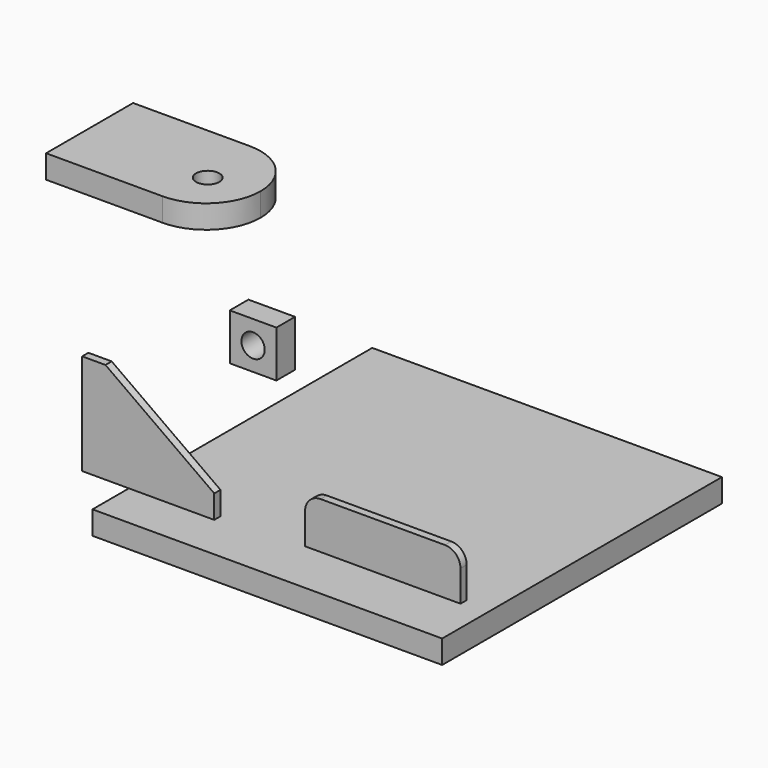
from build123d import *

# Parameters (mm, degrees)
F1_DEPTH  = 6.35
F0_W      = 127
F0_H      = 38.1
F2_R      = 12.7
F3_W      = 285.75
F3_H      = 19.05
F4_DEPTH  = 285.75
F5_W      = 38.1
F5_H      = 38.1
F5_R      = 9.525
F6_DEPTH  = 19.05
F7_W      = 139.7
F7_H      = 19.05
F8_DEPTH  = 88.9
F9_R      = 9.525
F10_DEPTH = 25.4
F11_R     = 44.44999


# Not quite as in the source:
# - a fillet or chamfer is up to 0.001 mm smaller than in the source, because OpenCascade refuses the exact size


with BuildPart() as f1:
    # F0 (on Front) → F1 (new body)
    with BuildSketch(Plane.XZ):
        Polygon((-51.8936398988, 44.7870248234), (-70.9436398988, 44.7870248234), (-70.9436398988, -37.7629751766), (37.0063601012, -37.7629751766), (37.0063601012, -18.7129751766), align=None)
    extrude(amount=-F1_DEPTH)


with BuildPart() as f1b:
    # F0 (on Front) → F1, piece 2 (new body)
    with BuildSketch(Plane.XZ):
        with Locations((174.7370118499, -13.572396946)):
            Rectangle(F0_W, F0_H)
    extrude(amount=-F1_DEPTH)

    # F2
    f2_edges = [f1b.edges().sort_by_distance(p)[0] for p in [
        (238.237012, 3.175, 5.477603),
        (111.237012, 3.175, 5.477603),
    ]]
    fillet(f2_edges, radius=F2_R)


with BuildPart() as f4:
    # F3 (on Front) → F4 (new body)
    with BuildSketch(Plane.XZ):
        with Locations((80.3878121078, -72.0597802344)):
            Rectangle(F3_W, F3_H)
    extrude(amount=-F4_DEPTH)


with BuildPart() as f6:
    # F5 (on Front) → F6 (new body)
    with BuildSketch(Plane.XZ):
        with Locations((68.7398687005, 98.0453198674)):
            Rectangle(F5_W, F5_H)
        with Locations((68.7398687005, 98.0453198674)):
            Circle(F5_R, mode=Mode.SUBTRACT)
    extrude(amount=-F6_DEPTH)


with BuildPart() as f8:
    # F7 (on Front) → F8 (new body)
    with BuildSketch(Plane.XZ):
        with Locations((-30.56688793, 171.7939794795)):
            Rectangle(F7_W, F7_H)
    extrude(amount=-F8_DEPTH)

    # F9 (on face) → F10 (cut)
    with BuildSketch(Plane.XY.offset(181.3189794795)):
        with Locations((1.18311207, 38.1)):
            Circle(F9_R)
    extrude(amount=-F10_DEPTH, mode=Mode.SUBTRACT)

    # F11 (radius 44.45 in the source; OpenCascade refuses exactly that, so slightly less here)
    f11_edges = [f8.edges().sort_by_distance(p)[0] for p in [
        (39.283112, 0, 171.793979),
        (39.283112, 88.9, 171.793979),
    ]]
    fillet(f11_edges, radius=F11_R)


solid = Compound([f1.part, f1b.part, f4.part, f6.part, f8.part])
